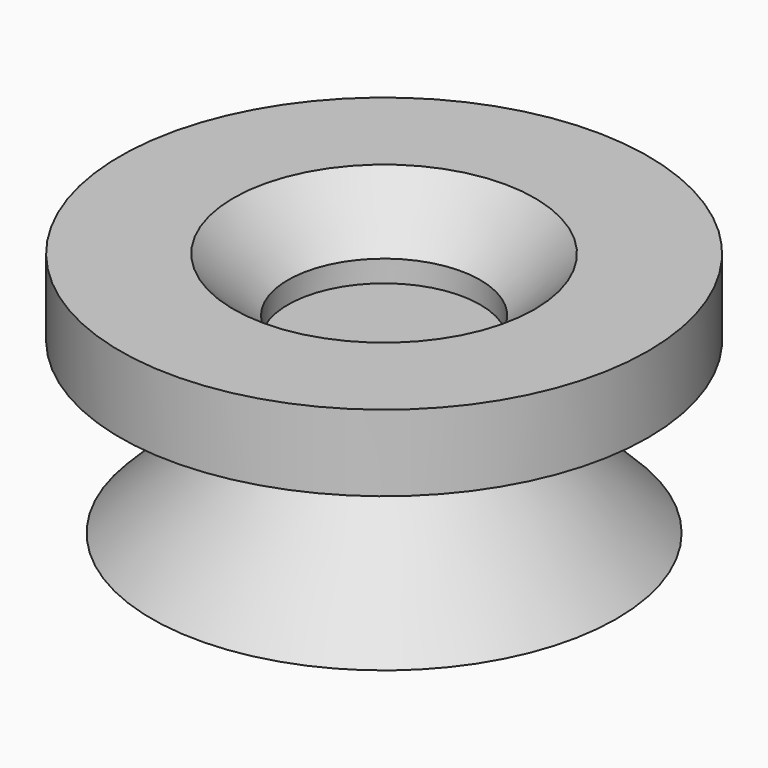
from build123d import *

# Parameters (mm, degrees)
F0_R     = 43.3405251853
F1_DEPTH = 25.4
F2_SIZE  = 25.39999
F3_DEPTH = 6.2703248113
F4_R     = 49.2381441728
F4_R_2   = 17.9405351853
F5_DEPTH = 14.2157543451
F6_SIZE  = 10.16


# Not quite as in the source:
# - a fillet or chamfer is up to 0.001 mm smaller than in the source, because OpenCascade refuses the exact size


with BuildPart() as f1:
    # F0 (on Top) → F1 (new body)
    with BuildSketch(Plane.XY):
        Circle(F0_R)
    extrude(amount=F1_DEPTH)

    # F2 (size 25.4 in the source; OpenCascade refuses exactly that, so slightly less here)
    f2_edges = [f1.edges().sort_by_distance(p)[0] for p in [
        (-43.340525, 0, 25.4),
    ]]
    chamfer(f2_edges, length=F2_SIZE)

    # F3 (add): a face of the model
    f3_faces = [f1.faces().sort_by_distance(p)[0] for p in [
        (0, 0, 25.4),
    ]]
    extrude(f3_faces, amount=F3_DEPTH)


with BuildPart() as f5:
    # F4 (on face) → F5 (new body)
    with BuildSketch(Plane.XY.offset(31.6703248113)):
        Circle(F4_R)
        Circle(F4_R_2, mode=Mode.SUBTRACT)
    extrude(amount=F5_DEPTH)

    # F6
    f6_edges = [f5.edges().sort_by_distance(p)[0] for p in [
        (-17.940535, 0, 45.886079),
    ]]
    chamfer(f6_edges, length=F6_SIZE)


solid = Compound([f1.part, f5.part])
